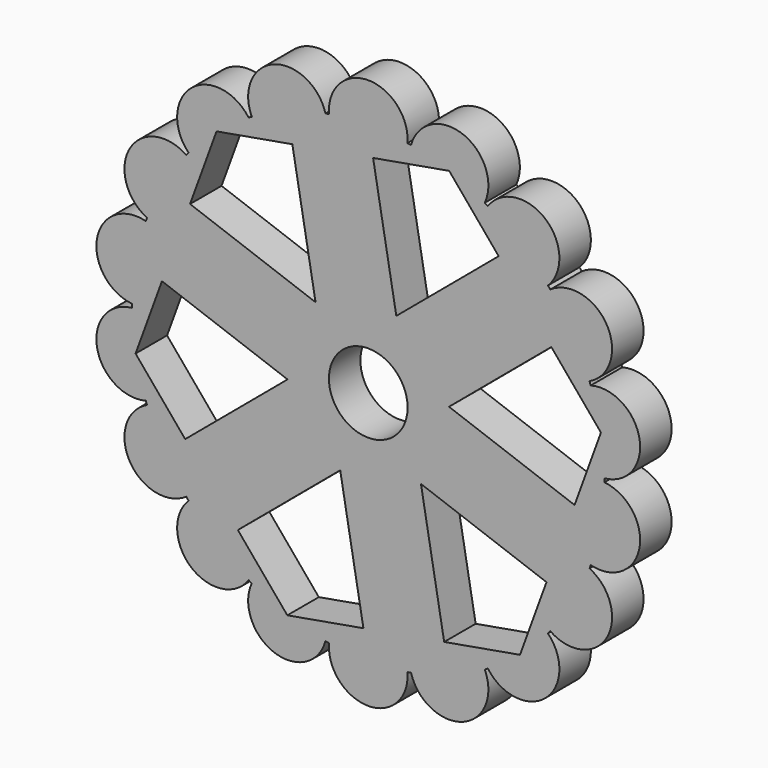
from build123d import *

# Parameters (mm, degrees)
F0_R     = 12.7
F1_DEPTH = 6.35


with BuildPart() as f1:
    # F0 (on Front) → F1 (new body, symmetric)
    with BuildSketch(Plane.XZ):
        with BuildLine():
            ThreePointArc((76.1977570212, -0.5846579641), (76.1994392532, -0.2923311333), (76.2, 0))
            ThreePointArc((76.2, 0), (76.1994392532, 0.2923311333), (76.1977570212, 0.5846579641))
            ThreePointArc((76.1977570212, 0.5846579641), (75.8897554045, 6.8691356552), (75.0643215302, 13.1067781397))
            Line((75.0643215302, 13.1067781397), (66.5824360485, -10.1528339917))
            Line((66.5824360485, -10.1528339917), (75.0423507795, -13.2319911382))
            ThreePointArc((75.0423507795, -13.2319911382), (75.8839990446, -6.9324374501), (76.1977570212, -0.5846579641))
        make_face()
        with BuildLine():
            ThreePointArc((75.0643215302, 13.1067781397), (75.8897554045, 6.8691356552), (76.1977570212, 0.5846579641))
            ThreePointArc((76.1977570212, 0.5846579641), (87.5494092428, 15.4373229946), (71.802434794, 25.5117690029))
            ThreePointArc((71.802434794, 25.5117690029), (73.6743133021, 19.4559903234), (75.0364186026, 13.2655901978))
            Line((75.0364186026, 13.2655901978), (75.0962151587, 13.1942390501))
            Line((75.0962151587, 13.1942390501), (75.0643215302, 13.1067781397))
        make_face()
        with BuildLine():
            ThreePointArc((71.802434794, -25.5117690029), (87.5494092428, -15.4373229946), (76.1977570212, -0.5846579641))
            ThreePointArc((76.1977570212, -0.5846579641), (75.8839990446, -6.9324374501), (75.0423507795, -13.2319911382))
            ThreePointArc((75.0423507795, -13.2319911382), (73.6786671882, -19.4394959134), (71.802434794, -25.5117690029))
        make_face()
        with BuildLine():
            ThreePointArc((75.0364186026, 13.2655901978), (73.6743133021, 19.4559903234), (71.802434794, 25.5117690029))
            ThreePointArc((71.802434794, 25.5117690029), (71.6045777039, 26.0619349214), (71.4025051926, 26.6105665521))
            ThreePointArc((71.4025051926, 26.6105665521), (68.9366006876, 32.4682165453), (65.9911357684, 38.1))
            Line((65.9911357684, 38.1), (59.08217806, 32.3026961351))
            Line((59.08217806, 32.3026961351), (75.0364186026, 13.2655901978))
        make_face()
        with BuildLine():
            ThreePointArc((71.802434794, -25.5117690029), (73.6786671882, -19.4394959134), (75.0423507795, -13.2319911382))
            Line((75.0423507795, -13.2319911382), (66.5824360485, -10.1528339917))
            Line((66.5824360485, -10.1528339917), (57.5160444937, -35.0153190433))
            Line((57.5160444937, -35.0153190433), (65.9911357684, -38.1))
            ThreePointArc((65.9911357684, -38.1), (68.9366006876, -32.4682165453), (71.4025051926, -26.6105665521))
            ThreePointArc((71.4025051926, -26.6105665521), (71.6045777039, -26.0619349214), (71.802434794, -25.5117690029))
        make_face()
        Polygon((57.5160444937, -35.0153190433), (66.5824360485, -10.1528339917), (26.0619349214, 4.5954222961), (59.08217806, 32.3026961351), (42.0838301815, 52.585664068), (9.0512150112, 24.8680088618), (1.5661335663, 67.3180151784), (-24.498605867, 62.7384980597), (-17.0107199103, 20.2725865657), (-57.5160444937, 35.0153190433), (-66.5824360485, 10.1528339917), (-26.0619349214, -4.5954222961), (-59.08217806, -32.3026961351), (-42.0838301815, -52.585664068), (-9.0512150112, -24.8680088618), (-1.5661335663, -67.3180151784), (24.498605867, -62.7384980597), (17.0107199103, -20.2725865657), align=None)
        Polygon((9.1694975967, 24.5029696394), (25.8049429742, 4.310466961), (16.6354453775, -20.1925026784), (-9.1694975967, -24.5029696394), (-25.8049429742, -4.310466961), (-16.6354453775, 20.1925026784), align=None, mode=Mode.SUBTRACT)
        with BuildLine():
            ThreePointArc((65.9911357684, 38.1), (68.9366006876, 32.4682165453), (71.4025051926, 26.6105665521))
            ThreePointArc((71.4025051926, 26.6105665521), (76.9896583964, 44.45), (58.7466792395, 48.5311001146))
            ThreePointArc((58.7466792395, 48.5311001146), (62.5866006876, 43.4667391734), (65.9911357684, 38.1))
        make_face()
        with BuildLine():
            ThreePointArc((58.7466792395, -48.5311001146), (76.9896583964, -44.45), (71.4025051926, -26.6105665521))
            ThreePointArc((71.4025051926, -26.6105665521), (68.9366006876, -32.4682165453), (65.9911357684, -38.1))
            ThreePointArc((65.9911357684, -38.1), (62.5866006876, -43.4667391734), (58.7466792395, -48.5311001146))
        make_face()
        with BuildLine():
            Line((42.0838301815, 52.585664068), (59.08217806, 32.3026961351))
            Line((59.08217806, 32.3026961351), (65.9911357684, 38.1))
            ThreePointArc((65.9911357684, 38.1), (62.5866006876, 43.4667391734), (58.7466792395, 48.5311001146))
            ThreePointArc((58.7466792395, 48.5311001146), (58.3725865657, 48.9804158581), (57.995057449, 49.4268480837))
            ThreePointArc((57.995057449, 49.4268480837), (53.6744308919, 54.0878495453), (48.9804158581, 58.3725865657))
            Line((48.9804158581, 58.3725865657), (42.0838301815, 52.585664068))
        make_face()
        with BuildLine():
            Line((65.9911357684, -38.1), (57.5160444937, -35.0153190433))
            Line((57.5160444937, -35.0153190433), (49.0065474088, -58.35064962))
            ThreePointArc((49.0065474088, -58.35064962), (53.6865385269, -54.0758317643), (57.995057449, -49.4268480837))
            ThreePointArc((57.995057449, -49.4268480837), (58.3725865657, -48.9804158581), (58.7466792395, -48.5311001146))
            ThreePointArc((58.7466792395, -48.5311001146), (62.5866006876, -43.4667391734), (65.9911357684, -38.1))
        make_face()
        with BuildLine():
            Line((26.1813579343, 71.5609984329), (42.0838301815, 52.585664068))
            Line((42.0838301815, 52.585664068), (48.9804158581, 58.3725865657))
            ThreePointArc((48.9804158581, 58.3725865657), (43.9456664643, 62.2512521883), (38.6052071601, 65.6968643097))
            ThreePointArc((38.6052071601, 65.6968643097), (38.1, 65.9911357684), (37.5925498612, 66.2815222738))
            ThreePointArc((37.5925498612, 66.2815222738), (31.9960317228, 69.1570238949), (26.1813579343, 71.5609984329))
        make_face()
        with BuildLine():
            ThreePointArc((57.995057449, -49.4268480837), (53.6865385269, -54.0758317643), (49.0065474088, -58.35064962))
            Line((49.0065474088, -58.35064962), (48.9746537804, -58.4381105304))
            Line((48.9746537804, -58.4381105304), (48.8829635959, -58.4542202932))
            ThreePointArc((48.8829635959, -58.4542202932), (43.8937236817, -62.2878882397), (38.6052071601, -65.6968643097))
            ThreePointArc((38.6052071601, -65.6968643097), (57.1438185011, -68.1013509933), (57.995057449, -49.4268480837))
        make_face()
        with BuildLine():
            ThreePointArc((48.9804158581, 58.3725865657), (53.6744308919, 54.0878495453), (57.995057449, 49.4268480837))
            ThreePointArc((57.995057449, 49.4268480837), (57.1438185011, 68.1013509933), (38.6052071601, 65.6968643097))
            ThreePointArc((38.6052071601, 65.6968643097), (43.9456664643, 62.2512521883), (48.9804158581, 58.3725865657))
        make_face()
        with BuildLine():
            Line((26.1215613783, 71.6323495805), (26.1813579343, 71.5609984329))
            ThreePointArc((26.1813579343, 71.5609984329), (31.9960317228, 69.1570238949), (37.5925498612, 66.2815222738))
            ThreePointArc((37.5925498612, 66.2815222738), (30.4055907417, 83.5386739879), (13.807377345, 74.9386170866))
            ThreePointArc((13.807377345, 74.9386170866), (19.9877747752, 73.5318220877), (26.0298711938, 71.6162398177))
            Line((26.0298711938, 71.6162398177), (26.1215613783, 71.6323495805))
        make_face()
        with BuildLine():
            ThreePointArc((38.6052071601, -65.6968643097), (43.8937236817, -62.2878882397), (48.8829635959, -58.4542202932))
            Line((48.8829635959, -58.4542202932), (24.498605867, -62.7384980597))
            Line((24.498605867, -62.7384980597), (26.0619349214, -71.6045777039))
            ThreePointArc((26.0619349214, -71.6045777039), (31.9383325803, -69.1836896384), (37.5925498612, -66.2815222738))
            ThreePointArc((37.5925498612, -66.2815222738), (38.1, -65.9911357684), (38.6052071601, -65.6968643097))
        make_face()
        with BuildLine():
            Line((26.0619349214, -71.6045777039), (24.498605867, -62.7384980597))
            Line((24.498605867, -62.7384980597), (-1.5661335663, -67.3180151784))
            Line((-1.5661335663, -67.3180151784), (0, -76.2))
            ThreePointArc((0, -76.2), (6.35, -75.9349557187), (12.6558259531, -75.1416666667))
            ThreePointArc((12.6558259531, -75.1416666667), (13.2319911382, -75.0423507795), (13.807377345, -74.9386170866))
            ThreePointArc((13.807377345, -74.9386170866), (20.0042362963, -73.5273454587), (26.0619349214, -71.6045777039))
        make_face()
        with BuildLine():
            Line((1.5661335663, 67.3180151784), (26.0298711938, 71.6162398177))
            ThreePointArc((26.0298711938, 71.6162398177), (19.9877747752, 73.5318220877), (13.807377345, 74.9386170866))
            ThreePointArc((13.807377345, 74.9386170866), (13.2319911382, 75.0423507795), (12.6558259531, 75.1416666667))
            ThreePointArc((12.6558259531, 75.1416666667), (6.35, 75.9349557187), (0, 76.2))
            Line((0, 76.2), (1.5661335663, 67.3180151784))
        make_face()
        with BuildLine():
            Line((-24.498605867, 62.7384980597), (1.5661335663, 67.3180151784))
            Line((1.5661335663, 67.3180151784), (0, 76.2))
            ThreePointArc((0, 76.2), (-6.35, 75.9349557187), (-12.6558259531, 75.1416666667))
            ThreePointArc((-12.6558259531, 75.1416666667), (-13.2319911382, 75.0423507795), (-13.807377345, 74.9386170866))
            ThreePointArc((-13.807377345, 74.9386170866), (-20.0042362963, 73.5273454587), (-26.0619349214, 71.6045777039))
            Line((-26.0619349214, 71.6045777039), (-24.498605867, 62.7384980597))
        make_face()
        with BuildLine():
            Line((0, -76.2), (-1.5661335663, -67.3180151784))
            Line((-1.5661335663, -67.3180151784), (-26.0298711938, -71.6162398177))
            ThreePointArc((-26.0298711938, -71.6162398177), (-19.9877747752, -73.5318220877), (-13.807377345, -74.9386170866))
            ThreePointArc((-13.807377345, -74.9386170866), (-13.2319911382, -75.0423507795), (-12.6558259531, -75.1416666667))
            ThreePointArc((-12.6558259531, -75.1416666667), (-6.35, -75.9349557187), (0, -76.2))
        make_face()
        with BuildLine():
            ThreePointArc((37.5925498612, -66.2815222738), (31.9383325803, -69.1836896384), (26.0619349214, -71.6045777039))
            ThreePointArc((26.0619349214, -71.6045777039), (20.0042362963, -73.5273454587), (13.807377345, -74.9386170866))
            ThreePointArc((13.807377345, -74.9386170866), (30.4055907417, -83.5386739879), (37.5925498612, -66.2815222738))
        make_face()
        with BuildLine():
            Line((-48.8829635959, 58.4542202932), (-24.498605867, 62.7384980597))
            Line((-24.498605867, 62.7384980597), (-26.0619349214, 71.6045777039))
            ThreePointArc((-26.0619349214, 71.6045777039), (-31.9383325803, 69.1836896384), (-37.5925498612, 66.2815222738))
            ThreePointArc((-37.5925498612, 66.2815222738), (-38.1, 65.9911357684), (-38.6052071601, 65.6968643097))
            ThreePointArc((-38.6052071601, 65.6968643097), (-43.8937236817, 62.2878882397), (-48.8829635959, 58.4542202932))
        make_face()
        with BuildLine():
            ThreePointArc((-12.6558259531, 75.1416666667), (-6.35, 75.9349557187), (0, 76.2))
            ThreePointArc((0, 76.2), (6.35, 75.9349557187), (12.6558259531, 75.1416666667))
            ThreePointArc((12.6558259531, 75.1416666667), (0, 88.9), (-12.6558259531, 75.1416666667))
        make_face()
        with BuildLine():
            ThreePointArc((-13.807377345, -74.9386170866), (-19.9877747752, -73.5318220877), (-26.0298711938, -71.6162398177))
            Line((-26.0298711938, -71.6162398177), (-26.1215613783, -71.6323495805))
            Line((-26.1215613783, -71.6323495805), (-26.1813579343, -71.5609984329))
            ThreePointArc((-26.1813579343, -71.5609984329), (-31.9960317228, -69.1570238949), (-37.5925498612, -66.2815222738))
            ThreePointArc((-37.5925498612, -66.2815222738), (-30.4055907417, -83.5386739879), (-13.807377345, -74.9386170866))
        make_face()
        with BuildLine():
            ThreePointArc((12.6558259531, -75.1416666667), (6.35, -75.9349557187), (0, -76.2))
            ThreePointArc((0, -76.2), (-6.35, -75.9349557187), (-12.6558259531, -75.1416666667))
            ThreePointArc((-12.6558259531, -75.1416666667), (0, -88.9), (12.6558259531, -75.1416666667))
        make_face()
        with BuildLine():
            Line((-48.9746537804, 58.4381105304), (-48.8829635959, 58.4542202932))
            ThreePointArc((-48.8829635959, 58.4542202932), (-43.8937236817, 62.2878882397), (-38.6052071601, 65.6968643097))
            ThreePointArc((-38.6052071601, 65.6968643097), (-57.1438185011, 68.1013509933), (-57.995057449, 49.4268480837))
            ThreePointArc((-57.995057449, 49.4268480837), (-53.6865385269, 54.0758317643), (-49.0065474088, 58.35064962))
            Line((-49.0065474088, 58.35064962), (-48.9746537804, 58.4381105304))
        make_face()
        with BuildLine():
            ThreePointArc((-37.5925498612, 66.2815222738), (-31.9383325803, 69.1836896384), (-26.0619349214, 71.6045777039))
            ThreePointArc((-26.0619349214, 71.6045777039), (-20.0042362963, 73.5273454587), (-13.807377345, 74.9386170866))
            ThreePointArc((-13.807377345, 74.9386170866), (-30.4055907417, 83.5386739879), (-37.5925498612, 66.2815222738))
        make_face()
        with BuildLine():
            ThreePointArc((-37.5925498612, -66.2815222738), (-31.9960317228, -69.1570238949), (-26.1813579343, -71.5609984329))
            Line((-26.1813579343, -71.5609984329), (-42.0838301815, -52.585664068))
            Line((-42.0838301815, -52.585664068), (-48.9804158581, -58.3725865657))
            ThreePointArc((-48.9804158581, -58.3725865657), (-43.9456664643, -62.2512521883), (-38.6052071601, -65.6968643097))
            ThreePointArc((-38.6052071601, -65.6968643097), (-38.1, -65.9911357684), (-37.5925498612, -66.2815222738))
        make_face()
        with BuildLine():
            Line((-48.9804158581, -58.3725865657), (-42.0838301815, -52.585664068))
            Line((-42.0838301815, -52.585664068), (-59.08217806, -32.3026961351))
            Line((-59.08217806, -32.3026961351), (-65.9911357684, -38.1))
            ThreePointArc((-65.9911357684, -38.1), (-62.5866006876, -43.4667391734), (-58.7466792395, -48.5311001146))
            ThreePointArc((-58.7466792395, -48.5311001146), (-58.3725865657, -48.9804158581), (-57.995057449, -49.4268480837))
            ThreePointArc((-57.995057449, -49.4268480837), (-53.6744308919, -54.0878495453), (-48.9804158581, -58.3725865657))
        make_face()
        with BuildLine():
            Line((-57.5160444937, 35.0153190433), (-49.0065474088, 58.35064962))
            ThreePointArc((-49.0065474088, 58.35064962), (-53.6865385269, 54.0758317643), (-57.995057449, 49.4268480837))
            ThreePointArc((-57.995057449, 49.4268480837), (-58.3725865657, 48.9804158581), (-58.7466792395, 48.5311001146))
            ThreePointArc((-58.7466792395, 48.5311001146), (-62.5866006876, 43.4667391734), (-65.9911357684, 38.1))
            Line((-65.9911357684, 38.1), (-57.5160444937, 35.0153190433))
        make_face()
        with BuildLine():
            Line((-66.5824360485, 10.1528339917), (-57.5160444937, 35.0153190433))
            Line((-57.5160444937, 35.0153190433), (-65.9911357684, 38.1))
            ThreePointArc((-65.9911357684, 38.1), (-68.9366006876, 32.4682165453), (-71.4025051926, 26.6105665521))
            ThreePointArc((-71.4025051926, 26.6105665521), (-71.6045777039, 26.0619349214), (-71.802434794, 25.5117690029))
            ThreePointArc((-71.802434794, 25.5117690029), (-73.6786671882, 19.4394959134), (-75.0423507795, 13.2319911382))
            Line((-75.0423507795, 13.2319911382), (-66.5824360485, 10.1528339917))
        make_face()
        with BuildLine():
            Line((-65.9911357684, -38.1), (-59.08217806, -32.3026961351))
            Line((-59.08217806, -32.3026961351), (-75.0364186026, -13.2655901978))
            ThreePointArc((-75.0364186026, -13.2655901978), (-73.6743133021, -19.4559903234), (-71.802434794, -25.5117690029))
            ThreePointArc((-71.802434794, -25.5117690029), (-71.6045777039, -26.0619349214), (-71.4025051926, -26.6105665521))
            ThreePointArc((-71.4025051926, -26.6105665521), (-68.9366006876, -32.4682165453), (-65.9911357684, -38.1))
        make_face()
        with BuildLine():
            ThreePointArc((-38.6052071601, -65.6968643097), (-43.9456664643, -62.2512521883), (-48.9804158581, -58.3725865657))
            ThreePointArc((-48.9804158581, -58.3725865657), (-53.6744308919, -54.0878495453), (-57.995057449, -49.4268480837))
            ThreePointArc((-57.995057449, -49.4268480837), (-57.1438185011, -68.1013509933), (-38.6052071601, -65.6968643097))
        make_face()
        with BuildLine():
            Line((-75.0643215302, -13.1067781397), (-66.5824360485, 10.1528339917))
            Line((-66.5824360485, 10.1528339917), (-75.0423507795, 13.2319911382))
            ThreePointArc((-75.0423507795, 13.2319911382), (-75.8839990446, 6.9324374501), (-76.1977570212, 0.5846579641))
            ThreePointArc((-76.1977570212, 0.5846579641), (-76.2, 0), (-76.1977570212, -0.5846579641))
            ThreePointArc((-76.1977570212, -0.5846579641), (-75.8897554045, -6.8691356552), (-75.0643215302, -13.1067781397))
        make_face()
        with BuildLine():
            ThreePointArc((-71.4025051926, 26.6105665521), (-68.9366006876, 32.4682165453), (-65.9911357684, 38.1))
            ThreePointArc((-65.9911357684, 38.1), (-62.5866006876, 43.4667391734), (-58.7466792395, 48.5311001146))
            ThreePointArc((-58.7466792395, 48.5311001146), (-76.9896583964, 44.45), (-71.4025051926, 26.6105665521))
        make_face()
        with BuildLine():
            ThreePointArc((-71.802434794, -25.5117690029), (-73.6743133021, -19.4559903234), (-75.0364186026, -13.2655901978))
            Line((-75.0364186026, -13.2655901978), (-75.0962151587, -13.1942390501))
            Line((-75.0962151587, -13.1942390501), (-75.0643215302, -13.1067781397))
            ThreePointArc((-75.0643215302, -13.1067781397), (-75.8897554045, -6.8691356552), (-76.1977570212, -0.5846579641))
            ThreePointArc((-76.1977570212, -0.5846579641), (-87.5494092428, -15.4373229946), (-71.802434794, -25.5117690029))
        make_face()
        with BuildLine():
            ThreePointArc((-58.7466792395, -48.5311001146), (-62.5866006876, -43.4667391734), (-65.9911357684, -38.1))
            ThreePointArc((-65.9911357684, -38.1), (-68.9366006876, -32.4682165453), (-71.4025051926, -26.6105665521))
            ThreePointArc((-71.4025051926, -26.6105665521), (-76.9896583964, -44.45), (-58.7466792395, -48.5311001146))
        make_face()
        with BuildLine():
            ThreePointArc((-76.1977570212, 0.5846579641), (-75.8839990446, 6.9324374501), (-75.0423507795, 13.2319911382))
            ThreePointArc((-75.0423507795, 13.2319911382), (-73.6786671882, 19.4394959134), (-71.802434794, 25.5117690029))
            ThreePointArc((-71.802434794, 25.5117690029), (-87.5494092428, 15.4373229946), (-76.1977570212, 0.5846579641))
        make_face()
        Polygon((16.6354453775, -20.1925026784), (25.8049429742, 4.310466961), (9.1694975967, 24.5029696394), (-16.6354453775, 20.1925026784), (-25.8049429742, -4.310466961), (-9.1694975967, -24.5029696394), align=None)
        Circle(F0_R, mode=Mode.SUBTRACT)
    extrude(amount=F1_DEPTH, both=True)


solid = f1.part
